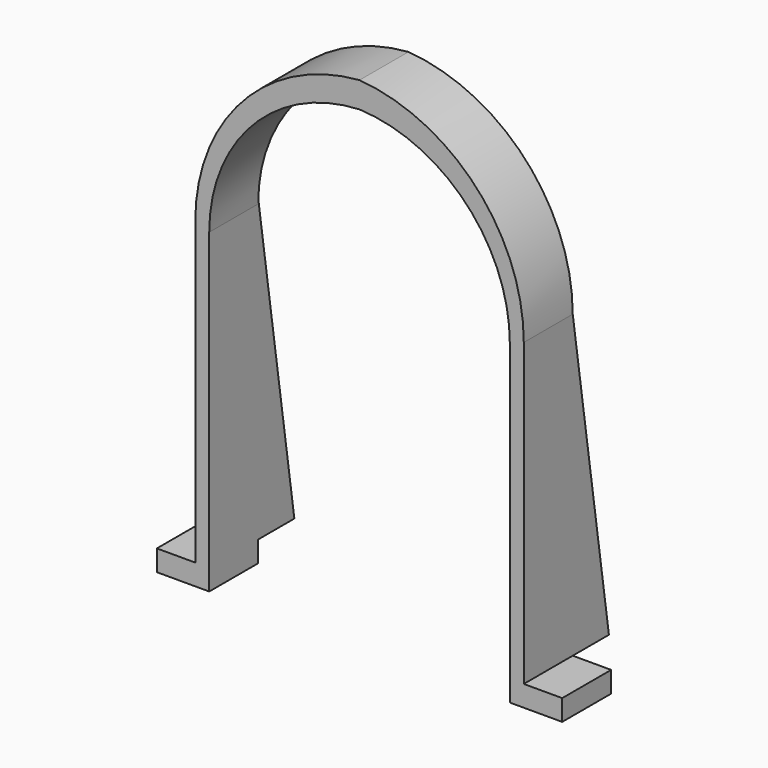
from build123d import *

# Parameters (mm, degrees)
F1_DEPTH    = 2.921
F3_DEPTH    = 5.842
F4_T1_DEPTH = 5.842
F5_T1_DEPTH = 90.842
F7_DEPTH    = 1.3335
F9_DEPTH    = 1.3335


# Not quite as in the source:
# - a fillet or chamfer that OpenCascade refuses, or shapes differently, is made with other operations: its cross-section is extruded or revolved along the edge and cut away or added


with BuildPart() as f1:
    # F0 (on Front) → F1 (new body, symmetric)
    with BuildSketch(Plane.XZ):
        Polygon((-14.351, -21.6027), (-14.351, 21.6027), (14.351, 21.6027), (14.351, -21.6027), (15.6845, -21.6027), (15.6845, 24.1027), (-15.6845, 24.1027), (-15.6845, -21.6027), align=None)
    extrude(amount=F1_DEPTH, both=True)

    # F2 (on face) → F3 (join, through all)
    with BuildSketch(Plane.XZ.offset(2.921)):
        Polygon((-14.351, -23.6027), (-14.351, -21.6027), (-15.6845, -21.6027), (-19.351, -21.6027), (-19.351, -23.6027), align=None)
        Polygon((15.6845, -21.6027), (14.351, -21.6027), (14.351, -23.6027), (19.351, -23.6027), (19.351, -21.6027), align=None)
    extrude(amount=-F3_DEPTH)

    # F4: fillet of radius 15 on 2 edges, made by hand

    # F4_s2 → F4_t1 (join)
    with BuildSketch(Plane.XZ.offset(-2.921)):
        with BuildLine():
            ThreePointArc((-14.351, 6.6027), (-9.9576017178, 17.2093017178), (0.649, 21.6027))
            Line((0.649, 21.6027), (-14.351, 21.6027))
            Line((-14.351, 21.6027), (-14.351, 6.6027))
        make_face()
        with BuildLine():
            ThreePointArc((14.351, 6.6027), (9.9576017178, 17.2093017178), (-0.649, 21.6027))
            Line((-0.649, 21.6027), (14.351, 21.6027))
            Line((14.351, 21.6027), (14.351, 6.6027))
        make_face()
    extrude(amount=F4_T1_DEPTH)

    # F5: fillet of radius 17 on 2 edges, made by hand

    # F5_s2 → F5_t1 (cut)
    with BuildSketch(Plane.XZ.offset(-45.421)):
        with BuildLine():
            ThreePointArc((1.3155, 24.1027), (-10.7053152802, 19.1235152802), (-15.6845, 7.1027))
            Line((-15.6845, 7.1027), (-15.6845, 24.1027))
            Line((-15.6845, 24.1027), (1.3155, 24.1027))
        make_face()
        with BuildLine():
            ThreePointArc((15.6845, 7.1027), (10.7053152802, 19.1235152802), (-1.3155, 24.1027))
            Line((-1.3155, 24.1027), (15.6845, 24.1027))
            Line((15.6845, 24.1027), (15.6845, 7.1027))
        make_face()
    extrude(amount=F5_T1_DEPTH, mode=Mode.SUBTRACT)

    # F6 (on face) → F7 (join, through all)
    with BuildSketch(Plane(origin=(-15.6845, 0, 0), x_dir=(0, -1, 0), z_dir=(-1, 0, 0))):
        Polygon((-2.921, -21.6027), (-2.921, 7.1027), (-7.239, -21.6027), align=None)
    extrude(amount=-F7_DEPTH)

    # F8 (on face) → F9 (join, through all)
    with BuildSketch(Plane.YZ.offset(15.6845)):
        Polygon((2.921, 6.6027), (2.921, -21.6027), (7.239, -21.6027), (2.921, 7.1027), align=None)
    extrude(amount=-F9_DEPTH)


solid = f1.part
